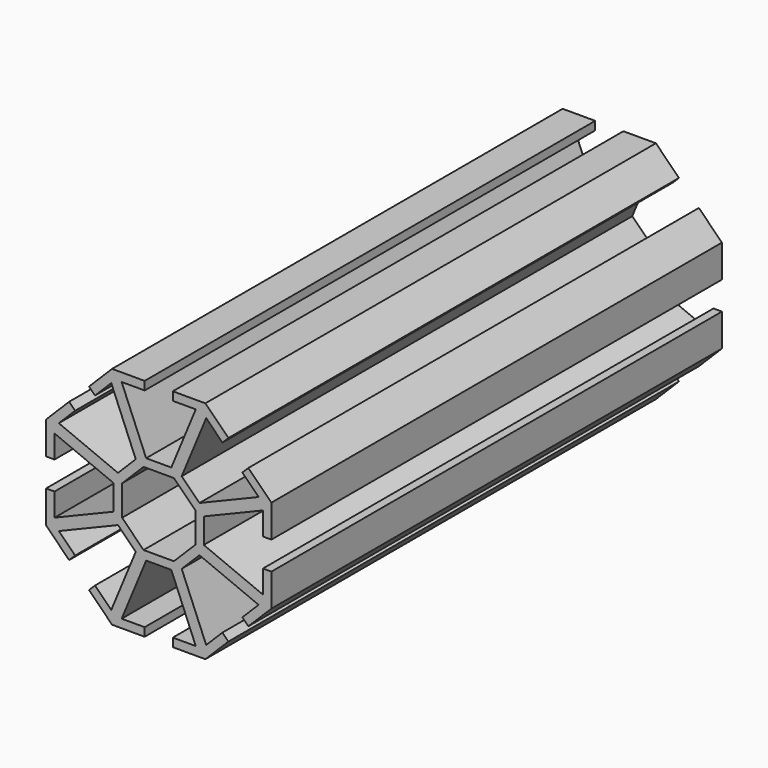
from build123d import *

# Parameters (mm, degrees)
F1_DEPTH        = 100
F3_DEPTH        = 100.001
F3_COPIES_COUNT = 8
F4_W            = 5
F4_H            = 1.5
F5_DEPTH        = 100.001
F5_COPIES_COUNT = 8


# Not quite as in the source:
# - a pattern or mirror of a feature is missing from the dataset's text; its kind, count and spacing are read off the source's solid


with BuildPart() as f1:
    # F0 (on Front) → F1 (new body)
    with BuildSketch(Plane.XZ):
        Polygon((8.2842712475, 20), (-8.2842712475, 20), (-20, 8.2842712475), (-20, -8.2842712475), (-8.2842712475, -20), (8.2842712475, -20), (20, -8.2842712475), (20, 8.2842712475), align=None)
        Polygon((-6.5, 2.6923881554), (-2.6923881554, 6.5), (2.6923881554, 6.5), (6.5, 2.6923881554), (6.5, -2.6923881554), (2.6923881554, -6.5), (-2.6923881554, -6.5), (-6.5, -2.6923881554), align=None, mode=Mode.SUBTRACT)
    extrude(amount=F1_DEPTH)

    # F2 (on face) → F3 (cut, through all)
    with BuildSketch(Plane.XZ.offset(100)):
        Polygon((-6.5805587036, 18.5), (-2.2313162987, 8), (2.2313162987, 8), (6.5805587036, 18.5), align=None)
    f3 = extrude(amount=-F3_DEPTH, mode=Mode.SUBTRACT)

    # F3_copies: F3 ×8 about axis
    f3_copies_axis = Axis((0, 0, 0), (0, 1, 0))
    for i in range(1, F3_COPIES_COUNT):
        add(f3.rotate(f3_copies_axis, i * 360 / F3_COPIES_COUNT), mode=Mode.SUBTRACT)

    # F4 (on face) → F5 (cut, through all)
    with BuildSketch(Plane.XZ.offset(100)):
        with Locations((0, 19.25)):
            Rectangle(F4_W, F4_H)
    f5 = extrude(amount=-F5_DEPTH, mode=Mode.SUBTRACT)

    # F5_copies: F5 ×8 about axis
    f5_copies_axis = Axis((0, 0, 0), (0, 1, 0))
    for i in range(1, F5_COPIES_COUNT):
        add(f5.rotate(f5_copies_axis, i * 360 / F5_COPIES_COUNT), mode=Mode.SUBTRACT)


solid = f1.part
